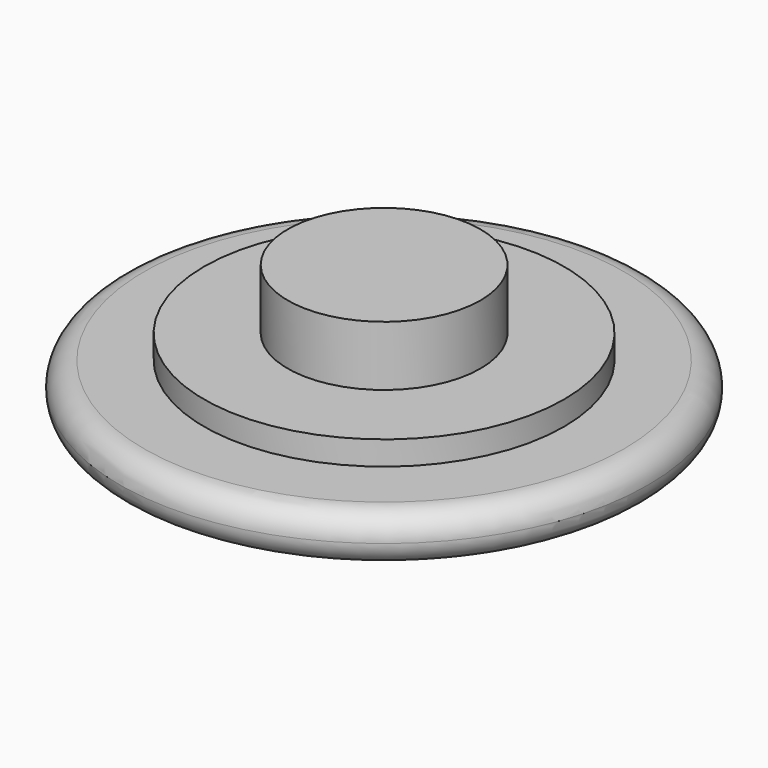
from build123d import *

# Parameters (mm, degrees)
F0_R     = 11
F0_R_2   = 7.5
F1_DEPTH = 2
F0_R_3   = 4.0165
F2_DEPTH = 3
F3_DEPTH = 5.5
F4_R     = 0.99999


# Not quite as in the source:
# - a fillet or chamfer is up to 0.001 mm smaller than in the source, because OpenCascade refuses the exact size


with BuildPart() as f1:
    # F0 (on Top) → F1 (new body)
    with BuildSketch(Plane.XY):
        Circle(F0_R)
        Circle(F0_R_2, mode=Mode.SUBTRACT)
    extrude(amount=F1_DEPTH)

    # F0 (on Top) → F2 (join)
    with BuildSketch(Plane.XY):
        Circle(F0_R_2)
        Circle(F0_R_3, mode=Mode.SUBTRACT)
    extrude(amount=F2_DEPTH)

    # F0 (on Top) → F3 (join)
    with BuildSketch(Plane.XY):
        Circle(F0_R_3)
    extrude(amount=F3_DEPTH)

    # F4 (radius 1 in the source; OpenCascade refuses exactly that, so slightly less here)
    f4_edges = [f1.edges().sort_by_distance(p)[0] for p in [
        (-11, 0, 2),
        (-11, 0, 0),
    ]]
    fillet(f4_edges, radius=F4_R)


solid = f1.part
